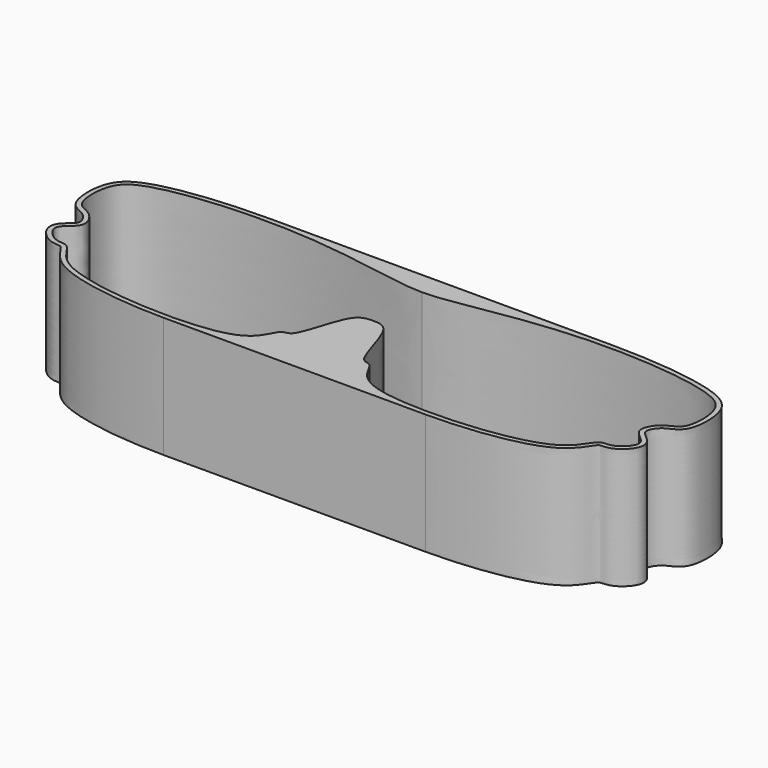
from build123d import *

# Parameters (mm, degrees)
F1_DEPTH = 30


# Not quite as in the source:
# - ends of sketch curves that miss each other by under 0.0002 mm in the source are joined
# - the dataset's text gives a spline's control points without its knots; the knots are read off the source's solid


with BuildPart() as f1:
    # F0 (on Top) → F1 (new body)
    with BuildSketch(Plane.XY):
        with BuildLine():
            add(Edge.make_bspline(
                [(-42.395039408, 22.1304505204), (-43.6521483854, 22.1319939219), (-46.7200481414, 22.0965925064), (-51.5392565596, 21.8940031156), (-56.6805860288, 21.4825365117), (-61.4565864596, 20.8910572441), (-65.0142175909, 20.2517015393), (-67.540161595, 19.6518866621), (-69.2599661497, 19.1561876348), (-70.7904208582, 18.6120117515), (-72.1270119472, 18.009117671), (-73.2907488927, 17.3201946709), (-74.2885497619, 16.5201472652), (-75.1153506877, 15.5942989885), (-75.9801519628, 14.1999293104), (-76.6411013247, 12.1929358894), (-76.917844612, 9.8659422384), (-76.9086445561, 7.9953923506), (-76.7804263202, 6.6313287436), (-76.5639298292, 5.561247128), (-76.3128381765, 4.761684668), (-76.0793783357, 4.1937473334), (-75.7927312767, 3.6606291479), (-75.4362787095, 3.1705419272), (-75.0400062235, 2.765315929), (-74.48370856, 2.324786982), (-73.7889147822, 1.9355309111), (-73.0347009974, 1.5882876142), (-72.4859881437, 1.3095804291), (-72.0905897437, 1.0566715157), (-71.714726824, 0.7676548096), (-71.2314411992, 0.2879331585), (-70.7360484653, -0.3916714763), (-70.4472988045, -0.9792350548), (-70.3136917269, -1.4126087035), (-70.2628727914, -1.7062742241), (-70.2576040022, -1.9568017588), (-70.2908169676, -2.1622595923), (-70.348936259, -2.3234807109), (-70.4756702849, -2.5398138532), (-70.6812361174, -2.7954999317), (-71.0496706434, -3.1733255714), (-71.5284480904, -3.5873386107), (-72.0495885767, -4.0398379696), (-72.4462223085, -4.4077501963), (-72.8333743415, -4.8182406815), (-73.1926728032, -5.2937194865), (-73.4422363204, -5.7697972276), (-73.5820305827, -6.2057841854), (-73.667248711, -6.6750796577), (-73.6583170163, -7.2442280542), (-73.5160096355, -7.8789091786), (-73.2793761342, -8.4647888496), (-72.8689534841, -9.1912246227), (-72.2150747915, -10.0102682772), (-71.437068551, -10.7110853472), (-70.7668255334, -11.1842012267), (-70.3311155094, -11.4387762102), (-69.9741144846, -11.613849399), (-69.6077581314, -11.7694328848), (-69.1584466117, -11.9140260964), (-68.6561511361, -12.0215111402), (-68.0476891617, -12.1039341838), (-67.5486591229, -12.1371349437), (-67.1865510652, -12.1798371859), (-66.9890765076, -12.2199936655), (-66.88432209, -12.2564127937), (-66.8230917264, -12.2863477416), (-66.772914702, -12.3163607967), (-66.6732450529, -12.3936082159), (-66.5051308104, -12.5691495886), (-66.301155477, -12.8260358832), (-65.9895848231, -13.2647010854), (-65.5284998757, -13.9653832257), (-64.8266133872, -14.9676825826), (-63.9207732102, -16.0579507121), (-62.9479775346, -16.9801256075), (-62.0149497845, -17.6904480234), (-61.2288653727, -18.2024662269), (-60.3677322518, -18.6796924304), (-59.1287915977, -19.2743252706), (-57.4168645857, -19.9465822961), (-55.1319851179, -20.6530842912), (-51.8213392178, -21.471017989), (-47.2736910167, -22.2726956469), (-41.4516729752, -22.903762178), (-36.4688659158, -23.1700526878), (-33.5418965798, -23.2113701207), (-32.5359604395, -23.2113692812)],
                knots=[0.1766200112, 0.1766200112, 0.1766200112, 0.1766200112, 0.1875, 0.203125, 0.21875, 0.234375, 0.25, 0.2578125, 0.265625, 0.2734375, 0.28125, 0.2890625, 0.296875, 0.3046875, 0.3125, 0.328125, 0.34375, 0.3515625, 0.359375, 0.3671875, 0.37109375, 0.375, 0.37890625, 0.3828125, 0.38671875, 0.390625, 0.3984375, 0.40625, 0.4140625, 0.41796875, 0.421875, 0.4296875, 0.4375, 0.4453125, 0.44921875, 0.453125, 0.45703125, 0.4609375, 0.46484375, 0.46875, 0.47265625, 0.4765625, 0.484375, 0.48828125, 0.4921875, 0.49609375, 0.5, 0.50390625, 0.505859375, 0.5078125, 0.51171875, 0.515625, 0.51953125, 0.5234375, 0.53125, 0.5390625, 0.54296875, 0.546875, 0.548828125, 0.55078125, 0.5546875, 0.55859375, 0.5625, 0.5703125, 0.57421875, 0.578125, 0.58203125, 0.583984375, 0.5859375, 0.58984375, 0.59375, 0.59765625, 0.6015625, 0.609375, 0.6171875, 0.625, 0.6328125, 0.63671875, 0.640625, 0.64453125, 0.6484375, 0.65625, 0.6640625, 0.671875, 0.6875, 0.703125, 0.71875, 0.7271730478, 0.7271730478, 0.7271730478, 0.7271730478], degree=3))
            add(Edge.make_bspline(
                [(-32.5359604395, -23.2113692812), (-31.6758556207, -23.2113685635), (-29.9120873457, -23.1893089136), (-27.3558590626, -23.0869341963), (-24.9019991381, -22.9091269156), (-22.6527377325, -22.6590788965), (-20.6468740684, -22.3358022077), (-18.8835769503, -21.9381454749), (-16.8183293919, -21.3053958059), (-15.1387331774, -20.5100405296), (-13.7819372426, -19.5425447913), (-12.9174022259, -18.7361896815), (-12.315497581, -18.0080720967), (-11.8962380792, -17.3972257139), (-11.523515163, -16.7912038109), (-11.1258969534, -16.0624123646), (-10.7883816101, -15.4308012957), (-10.5483676461, -15.0265890776), (-10.3867902249, -14.7868335879), (-10.253463351, -14.6239278354), (-10.1798775644, -14.5587218759), (-10.1623324279, -14.5472416405), (-10.157556386, -14.5443942619), (-10.1010062585, -14.5193724081), (-9.9237338661, -14.4745800811), (-9.6339783641, -14.41389781), (-9.2453733984, -14.3116388902), (-8.7838186544, -14.1237531909), (-8.3823605633, -13.8644826032), (-8.0799500073, -13.5949875264), (-7.7939062442, -13.2838623393), (-7.4959985315, -12.8624558318), (-7.1820200006, -12.3029222273), (-6.8924671342, -11.6874790116), (-6.5248609637, -10.7957447126), (-6.0856201466, -9.5607733896), (-5.5676376981, -7.9515296734), (-5.0465950473, -6.2946985681), (-4.5138317261, -4.6764434327), (-4.0558112809, -3.4367781242), (-3.6822211566, -2.560702725), (-3.4008437861, -1.9759785391), (-3.1213188068, -1.4769240618), (-2.856447289, -1.0866032187), (-2.6045553334, -0.7937104629), (-2.2809488422, -0.5002013352), (-1.8946316039, -0.2721449841), (-1.374196514, -0.1111220013), (-0.7456447191, -0.0337503318), (-0.2554461531, -0.0178101934), (5.68e-08, -0.0102657556)],
                knots=[0.7271730478, 0.7271730478, 0.7271730478, 0.7271730478, 0.734375, 0.7421875, 0.75, 0.7578125, 0.765625, 0.7734375, 0.78125, 0.796875, 0.8046875, 0.8125, 0.8203125, 0.82421875, 0.828125, 0.8359375, 0.84375, 0.84765625, 0.8515625, 0.85546875, 0.859375, 0.861328125, 0.86328125, 0.8671875, 0.87109375, 0.875, 0.87890625, 0.8828125, 0.88671875, 0.888671875, 0.890625, 0.89453125, 0.8984375, 0.90234375, 0.90625, 0.9140625, 0.921875, 0.9296875, 0.9375, 0.9453125, 0.94921875, 0.953125, 0.95703125, 0.9609375, 0.96484375, 0.96875, 0.9765625, 0.984375, 0.9921875, 0.9996578295, 0.9996578295, 0.9996578295, 0.9996578295], degree=3))
            add(Edge.make_bspline(
                [(32.5359604395, -23.2113692812), (31.6758556207, -23.2113685635), (29.9120873457, -23.1893089136), (27.3558590626, -23.0869341963), (24.9019991381, -22.9091269156), (22.6527377325, -22.6590788965), (20.6468740684, -22.3358022077), (18.8835769503, -21.9381454749), (16.8183293919, -21.3053958059), (15.1387331774, -20.5100405296), (13.7819372426, -19.5425447913), (12.9174022259, -18.7361896815), (12.315497581, -18.0080720967), (11.8962380792, -17.3972257139), (11.523515163, -16.7912038109), (11.1258969534, -16.0624123646), (10.7883816101, -15.4308012957), (10.5483676461, -15.0265890776), (10.3867902249, -14.7868335879), (10.253463351, -14.6239278354), (10.1798775644, -14.5587218759), (10.1623324279, -14.5472416405), (10.157556386, -14.5443942619), (10.1010062585, -14.5193724081), (9.9237338661, -14.4745800811), (9.6339783641, -14.41389781), (9.2453733984, -14.3116388902), (8.7838186544, -14.1237531909), (8.3823605633, -13.8644826032), (8.0799500073, -13.5949875264), (7.7939062442, -13.2838623393), (7.4959985315, -12.8624558318), (7.1820200006, -12.3029222273), (6.8924671342, -11.6874790116), (6.5248609637, -10.7957447126), (6.0856201466, -9.5607733896), (5.5676376981, -7.9515296734), (5.0465950473, -6.2946985681), (4.5138317261, -4.6764434327), (4.0558112809, -3.4367781242), (3.6822211566, -2.560702725), (3.4008437861, -1.9759785391), (3.1213188068, -1.4769240618), (2.856447289, -1.0866032187), (2.6045553334, -0.7937104629), (2.2809488422, -0.5002013352), (1.8946316039, -0.2721449841), (1.374196514, -0.1111220013), (0.7456447191, -0.0337503318), (0.2554461531, -0.0178101934), (5.68e-08, -0.0102657556)],
                knots=[0.7271730478, 0.7271730478, 0.7271730478, 0.7271730478, 0.734375, 0.7421875, 0.75, 0.7578125, 0.765625, 0.7734375, 0.78125, 0.796875, 0.8046875, 0.8125, 0.8203125, 0.82421875, 0.828125, 0.8359375, 0.84375, 0.84765625, 0.8515625, 0.85546875, 0.859375, 0.861328125, 0.86328125, 0.8671875, 0.87109375, 0.875, 0.87890625, 0.8828125, 0.88671875, 0.888671875, 0.890625, 0.89453125, 0.8984375, 0.90234375, 0.90625, 0.9140625, 0.921875, 0.9296875, 0.9375, 0.9453125, 0.94921875, 0.953125, 0.95703125, 0.9609375, 0.96484375, 0.96875, 0.9765625, 0.984375, 0.9921875, 0.9996578295, 0.9996578295, 0.9996578295, 0.9996578295], degree=3))
            add(Edge.make_bspline(
                [(42.395039408, 22.1304505204), (43.6521483854, 22.1319939219), (46.7200481414, 22.0965925064), (51.5392565596, 21.8940031156), (56.6805860288, 21.4825365117), (61.4565864596, 20.8910572441), (65.0142175909, 20.2517015393), (67.540161595, 19.6518866621), (69.2599661497, 19.1561876348), (70.7904208582, 18.6120117515), (72.1270119472, 18.009117671), (73.2907488927, 17.3201946709), (74.2885497619, 16.5201472652), (75.1153506877, 15.5942989885), (75.9801519628, 14.1999293104), (76.6411013247, 12.1929358894), (76.917844612, 9.8659422384), (76.9086445561, 7.9953923506), (76.7804263202, 6.6313287436), (76.5639298292, 5.561247128), (76.3128381765, 4.761684668), (76.0793783357, 4.1937473334), (75.7927312767, 3.6606291479), (75.4362787095, 3.1705419272), (75.0400062235, 2.765315929), (74.48370856, 2.324786982), (73.7889147822, 1.9355309111), (73.0347009974, 1.5882876142), (72.4859881437, 1.3095804291), (72.0905897437, 1.0566715157), (71.714726824, 0.7676548096), (71.2314411992, 0.2879331585), (70.7360484653, -0.3916714763), (70.4472988045, -0.9792350548), (70.3136917269, -1.4126087035), (70.2628727914, -1.7062742241), (70.2576040022, -1.9568017588), (70.2908169676, -2.1622595923), (70.348936259, -2.3234807109), (70.4756702849, -2.5398138532), (70.6812361174, -2.7954999317), (71.0496706434, -3.1733255714), (71.5284480904, -3.5873386107), (72.0495885767, -4.0398379696), (72.4462223085, -4.4077501963), (72.8333743415, -4.8182406815), (73.1926728032, -5.2937194865), (73.4422363204, -5.7697972276), (73.5820305827, -6.2057841854), (73.667248711, -6.6750796577), (73.6583170163, -7.2442280542), (73.5160096355, -7.8789091786), (73.2793761342, -8.4647888496), (72.8689534841, -9.1912246227), (72.2150747915, -10.0102682772), (71.437068551, -10.7110853472), (70.7668255334, -11.1842012267), (70.3311155094, -11.4387762102), (69.9741144846, -11.613849399), (69.6077581314, -11.7694328848), (69.1584466117, -11.9140260964), (68.6561511361, -12.0215111402), (68.0476891617, -12.1039341838), (67.5486591229, -12.1371349437), (67.1865510652, -12.1798371859), (66.9890765076, -12.2199936655), (66.88432209, -12.2564127937), (66.8230917264, -12.2863477416), (66.772914702, -12.3163607967), (66.6732450529, -12.3936082159), (66.5051308104, -12.5691495886), (66.301155477, -12.8260358832), (65.9895848231, -13.2647010854), (65.5284998757, -13.9653832257), (64.8266133872, -14.9676825826), (63.9207732102, -16.0579507121), (62.9479775346, -16.9801256075), (62.0149497845, -17.6904480234), (61.2288653727, -18.2024662269), (60.3677322518, -18.6796924304), (59.1287915977, -19.2743252706), (57.4168645857, -19.9465822961), (55.1319851179, -20.6530842912), (51.8213392178, -21.471017989), (47.2736910167, -22.2726956469), (41.4516729752, -22.903762178), (36.4688659158, -23.1700526878), (33.5418965798, -23.2113701207), (32.5359604395, -23.2113692812)],
                knots=[0.1766200112, 0.1766200112, 0.1766200112, 0.1766200112, 0.1875, 0.203125, 0.21875, 0.234375, 0.25, 0.2578125, 0.265625, 0.2734375, 0.28125, 0.2890625, 0.296875, 0.3046875, 0.3125, 0.328125, 0.34375, 0.3515625, 0.359375, 0.3671875, 0.37109375, 0.375, 0.37890625, 0.3828125, 0.38671875, 0.390625, 0.3984375, 0.40625, 0.4140625, 0.41796875, 0.421875, 0.4296875, 0.4375, 0.4453125, 0.44921875, 0.453125, 0.45703125, 0.4609375, 0.46484375, 0.46875, 0.47265625, 0.4765625, 0.484375, 0.48828125, 0.4921875, 0.49609375, 0.5, 0.50390625, 0.505859375, 0.5078125, 0.51171875, 0.515625, 0.51953125, 0.5234375, 0.53125, 0.5390625, 0.54296875, 0.546875, 0.548828125, 0.55078125, 0.5546875, 0.55859375, 0.5625, 0.5703125, 0.57421875, 0.578125, 0.58203125, 0.583984375, 0.5859375, 0.58984375, 0.59375, 0.59765625, 0.6015625, 0.609375, 0.6171875, 0.625, 0.6328125, 0.63671875, 0.640625, 0.64453125, 0.6484375, 0.65625, 0.6640625, 0.671875, 0.6875, 0.703125, 0.71875, 0.7271730478, 0.7271730478, 0.7271730478, 0.7271730478], degree=3))
            add(Edge.make_bspline(
                [(0, 17.6205115976), (0.6478802761, 17.6205115976), (1.9419420193, 17.6641721124), (4.037973266, 17.8605516244), (6.0389243133, 18.1345331493), (7.8613677003, 18.4192515273), (9.8576727195, 18.7479380209), (12.67286482, 19.2280616688), (16.5046638703, 19.8632696372), (20.7401720631, 20.5070177502), (25.3295252409, 21.1087700711), (30.2245515949, 21.6175981933), (35.3754389025, 21.9843653778), (39.4949880805, 22.1137618575), (41.8467855229, 22.1297774078), (42.395039408, 22.1304505204)],
                knots=[0, 0, 0, 0, 0.015625, 0.03125, 0.046875, 0.0546875, 0.0625, 0.078125, 0.09375, 0.109375, 0.125, 0.140625, 0.15625, 0.171875, 0.1766200112, 0.1766200112, 0.1766200112, 0.1766200112], degree=3))
            add(Edge.make_bspline(
                [(0, 17.6205115976), (-0.6478802761, 17.6205115976), (-1.9419420193, 17.6641721124), (-4.037973266, 17.8605516244), (-6.0389243133, 18.1345331493), (-7.8613677003, 18.4192515273), (-9.8576727195, 18.7479380209), (-12.67286482, 19.2280616688), (-16.5046638703, 19.8632696372), (-20.7401720631, 20.5070177502), (-25.3295252409, 21.1087700711), (-30.2245515949, 21.6175981933), (-35.3754389025, 21.9843653778), (-39.4949880805, 22.1137618575), (-41.8467855229, 22.1297774078), (-42.395039408, 22.1304505204)],
                knots=[0, 0, 0, 0, 0.015625, 0.03125, 0.046875, 0.0546875, 0.0625, 0.078125, 0.09375, 0.109375, 0.125, 0.140625, 0.15625, 0.171875, 0.1766200112, 0.1766200112, 0.1766200112, 0.1766200112], degree=3))
        make_face()
        with BuildLine():
            add(Edge.make_bspline(
                [(0, 16.420511597), (-2.4272201873, 16.4205115969), (-9.284878657, 17.2589122929), (-36.1073015385, 22.4659501127), (-70.1241556478, 19.5493275569), (-76.0996077571, 13.3535139167), (-75.7672673785, 3.1509984866), (-70.998464322, 2.7353495526), (-67.3901194658, -3.2263797531), (-74.5441430478, -6.0993995369), (-69.4013381825, -11.5019542975), (-65.3179114086, -10.2636553551), (-62.6521700492, -21.2501398582), (-21.7153914905, -23.5032808988), (-12.9520738609, -18.1044426924), (-11.2138304308, -12.8795020048), (-7.7287441661, -13.9019263951), (-5.1595610101, 1.0388377902), (-1.3702954023, 1.1500401483), (0, 1.1902537662)],
                knots=[0, 0, 0, 0, 0.0561924901, 0.1596924953, 0.2721112738, 0.3246180164, 0.3802739948, 0.419522857, 0.4630370663, 0.5067105017, 0.5504487633, 0.5851599221, 0.6396287773, 0.7605373505, 0.8221828526, 0.861431716, 0.889834155, 0.9601524079, 1, 1, 1, 1], degree=3))
            add(Edge.make_bspline(
                [(0, 16.420511597), (2.4272201873, 16.4205115969), (9.284878657, 17.2589122929), (36.1073015385, 22.4659501127), (70.1241556478, 19.5493275569), (76.0996077571, 13.3535139167), (75.7672673785, 3.1509984866), (70.998464322, 2.7353495526), (67.3901194658, -3.2263797531), (74.5441430478, -6.0993995369), (69.4013381825, -11.5019542975), (65.3179114086, -10.2636553551), (62.6521700492, -21.2501398582), (21.7153914905, -23.5032808988), (12.9520738609, -18.1044426924), (11.2138304308, -12.8795020048), (7.7287441661, -13.9019263951), (5.1595610101, 1.0388377902), (1.3702954023, 1.1500401483), (0, 1.1902537662)],
                knots=[0, 0, 0, 0, 0.0561924901, 0.1596924953, 0.2721112738, 0.3246180164, 0.3802739948, 0.419522857, 0.4630370663, 0.5067105017, 0.5504487633, 0.5851599221, 0.6396287773, 0.7605373505, 0.8221828526, 0.861431716, 0.889834155, 0.9601524079, 1, 1, 1, 1], degree=3))
        make_face(mode=Mode.SUBTRACT)
        with BuildLine():
            add(Edge.make_bspline(
                [(-32.5359604395, -23.2113692812), (-31.6758556207, -23.2113685635), (-29.9120873457, -23.1893089136), (-27.3558590626, -23.0869341963), (-24.9019991381, -22.9091269156), (-22.6527377325, -22.6590788965), (-20.6468740684, -22.3358022077), (-18.8835769503, -21.9381454749), (-16.8183293919, -21.3053958059), (-15.1387331774, -20.5100405296), (-13.7819372426, -19.5425447913), (-12.9174022259, -18.7361896815), (-12.315497581, -18.0080720967), (-11.8962380792, -17.3972257139), (-11.523515163, -16.7912038109), (-11.1258969534, -16.0624123646), (-10.7883816101, -15.4308012957), (-10.5483676461, -15.0265890776), (-10.3867902249, -14.7868335879), (-10.253463351, -14.6239278354), (-10.1798775644, -14.5587218759), (-10.1623324279, -14.5472416405), (-10.157556386, -14.5443942619), (-10.1010062585, -14.5193724081), (-9.9237338661, -14.4745800811), (-9.6339783641, -14.41389781), (-9.2453733984, -14.3116388902), (-8.7838186544, -14.1237531909), (-8.3823605633, -13.8644826032), (-8.0799500073, -13.5949875264), (-7.7939062442, -13.2838623393), (-7.4959985315, -12.8624558318), (-7.1820200006, -12.3029222273), (-6.8924671342, -11.6874790116), (-6.5248609637, -10.7957447126), (-6.0856201466, -9.5607733896), (-5.5676376981, -7.9515296734), (-5.0465950473, -6.2946985681), (-4.5138317261, -4.6764434327), (-4.0558112809, -3.4367781242), (-3.6822211566, -2.560702725), (-3.4008437861, -1.9759785391), (-3.1213188068, -1.4769240618), (-2.856447289, -1.0866032187), (-2.6045553334, -0.7937104629), (-2.2809488422, -0.5002013352), (-1.8946316039, -0.2721449841), (-1.374196514, -0.1111220013), (-0.7456447191, -0.0337503318), (-0.2554461531, -0.0178101934), (5.68e-08, -0.0102657556)],
                knots=[0.7271730478, 0.7271730478, 0.7271730478, 0.7271730478, 0.734375, 0.7421875, 0.75, 0.7578125, 0.765625, 0.7734375, 0.78125, 0.796875, 0.8046875, 0.8125, 0.8203125, 0.82421875, 0.828125, 0.8359375, 0.84375, 0.84765625, 0.8515625, 0.85546875, 0.859375, 0.861328125, 0.86328125, 0.8671875, 0.87109375, 0.875, 0.87890625, 0.8828125, 0.88671875, 0.888671875, 0.890625, 0.89453125, 0.8984375, 0.90234375, 0.90625, 0.9140625, 0.921875, 0.9296875, 0.9375, 0.9453125, 0.94921875, 0.953125, 0.95703125, 0.9609375, 0.96484375, 0.96875, 0.9765625, 0.984375, 0.9921875, 0.9996578295, 0.9996578295, 0.9996578295, 0.9996578295], degree=3))
            Line((-32.5359604395, -23.2113692812), (32.5359604395, -23.2113600024))
            add(Edge.make_bspline(
                [(32.5359604395, -23.2113600024), (31.6758556207, -23.2113685635), (29.9120873457, -23.1893089136), (27.3558590626, -23.0869341963), (24.9019991381, -22.9091269156), (22.6527377325, -22.6590788965), (20.6468740684, -22.3358022077), (18.8835769503, -21.9381454749), (16.8183293919, -21.3053958059), (15.1387331774, -20.5100405296), (13.7819372426, -19.5425447913), (12.9174022259, -18.7361896815), (12.315497581, -18.0080720967), (11.8962380792, -17.3972257139), (11.523515163, -16.7912038109), (11.1258969534, -16.0624123646), (10.7883816101, -15.4308012957), (10.5483676461, -15.0265890776), (10.3867902249, -14.7868335879), (10.253463351, -14.6239278354), (10.1798775644, -14.5587218759), (10.1623324279, -14.5472416405), (10.157556386, -14.5443942619), (10.1010062585, -14.5193724081), (9.9237338661, -14.4745800811), (9.6339783641, -14.41389781), (9.2453733984, -14.3116388902), (8.7838186544, -14.1237531909), (8.3823605633, -13.8644826032), (8.0799500073, -13.5949875264), (7.7939062442, -13.2838623393), (7.4959985315, -12.8624558318), (7.1820200006, -12.3029222273), (6.8924671342, -11.6874790116), (6.5248609637, -10.7957447126), (6.0856201466, -9.5607733896), (5.5676376981, -7.9515296734), (5.0465950473, -6.2946985681), (4.5138317261, -4.6764434327), (4.0558112809, -3.4367781242), (3.6822211566, -2.560702725), (3.4008437861, -1.9759785391), (3.1213188068, -1.4769240618), (2.856447289, -1.0866032187), (2.6045553334, -0.7937104629), (2.2809488422, -0.5002013352), (1.8946316039, -0.2721449841), (1.374196514, -0.1111220013), (0.7456447191, -0.0337503318), (0.2554461531, -0.0178101934), (5.68e-08, -0.0102657556)],
                knots=[0.7271730478, 0.7271730478, 0.7271730478, 0.7271730478, 0.734375, 0.7421875, 0.75, 0.7578125, 0.765625, 0.7734375, 0.78125, 0.796875, 0.8046875, 0.8125, 0.8203125, 0.82421875, 0.828125, 0.8359375, 0.84375, 0.84765625, 0.8515625, 0.85546875, 0.859375, 0.861328125, 0.86328125, 0.8671875, 0.87109375, 0.875, 0.87890625, 0.8828125, 0.88671875, 0.888671875, 0.890625, 0.89453125, 0.8984375, 0.90234375, 0.90625, 0.9140625, 0.921875, 0.9296875, 0.9375, 0.9453125, 0.94921875, 0.953125, 0.95703125, 0.9609375, 0.96484375, 0.96875, 0.9765625, 0.984375, 0.9921875, 0.9996578295, 0.9996578295, 0.9996578295, 0.9996578295], degree=3))
        make_face()
        with BuildLine():
            Line((42.395039408, 22.1304505204), (-42.395039408, 22.1304505204))
            add(Edge.make_bspline(
                [(0, 17.6205115976), (-0.6478802761, 17.6205115976), (-1.9419420193, 17.6641721124), (-4.037973266, 17.8605516244), (-6.0389243133, 18.1345331493), (-7.8613677003, 18.4192515273), (-9.8576727195, 18.7479380209), (-12.67286482, 19.2280616688), (-16.5046638703, 19.8632696372), (-20.7401720631, 20.5070177502), (-25.3295252409, 21.1087700711), (-30.2245515949, 21.6175981933), (-35.3754389025, 21.9843653778), (-39.4949880805, 22.1137618575), (-41.8467855229, 22.1297774078), (-42.395039408, 22.1304505204)],
                knots=[0, 0, 0, 0, 0.015625, 0.03125, 0.046875, 0.0546875, 0.0625, 0.078125, 0.09375, 0.109375, 0.125, 0.140625, 0.15625, 0.171875, 0.1766200112, 0.1766200112, 0.1766200112, 0.1766200112], degree=3))
            add(Edge.make_bspline(
                [(0, 17.6205115976), (0.6478802761, 17.6205115976), (1.9419420193, 17.6641721124), (4.037973266, 17.8605516244), (6.0389243133, 18.1345331493), (7.8613677003, 18.4192515273), (9.8576727195, 18.7479380209), (12.67286482, 19.2280616688), (16.5046638703, 19.8632696372), (20.7401720631, 20.5070177502), (25.3295252409, 21.1087700711), (30.2245515949, 21.6175981933), (35.3754389025, 21.9843653778), (39.4949880805, 22.1137618575), (41.8467855229, 22.1297774078), (42.395039408, 22.1304505204)],
                knots=[0, 0, 0, 0, 0.015625, 0.03125, 0.046875, 0.0546875, 0.0625, 0.078125, 0.09375, 0.109375, 0.125, 0.140625, 0.15625, 0.171875, 0.1766200112, 0.1766200112, 0.1766200112, 0.1766200112], degree=3))
        make_face()
    extrude(amount=F1_DEPTH)


solid = f1.part
